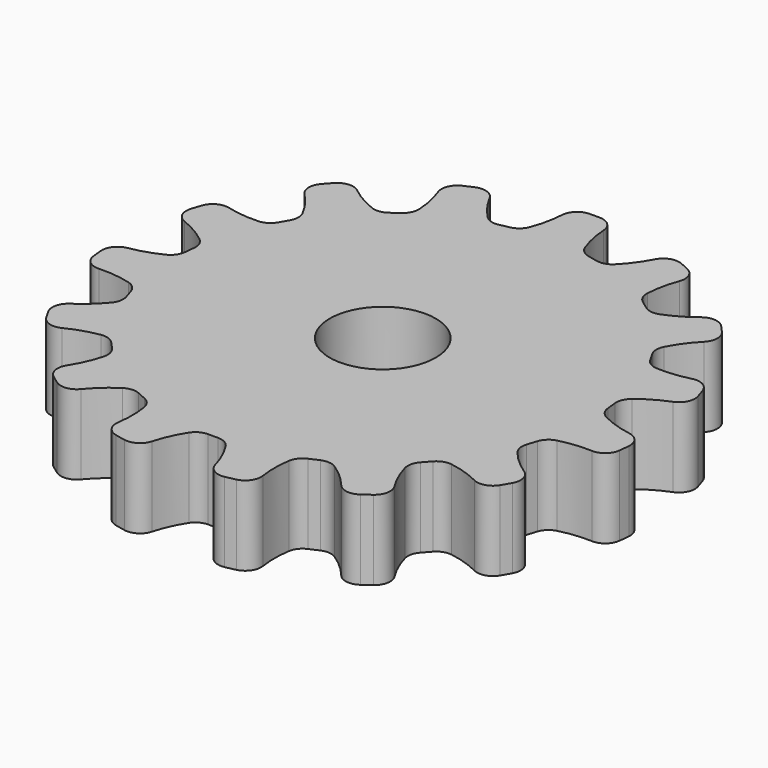
from build123d import *

# Parameters (mm, degrees)
F0_R            = 50
F1_DEPTH        = 15
F3_DEPTH        = 25
F3_COPIES_COUNT = 15
F4_R            = 3
F5_R            = 10
F6_DEPTH        = 25


# Not quite as in the source:
# - a pattern or mirror of a feature is missing from the dataset's text; its kind, count and spacing are read off the source's solid


with BuildPart() as f1:
    # F0 (on Top) → F1 (new body)
    with BuildSketch(Plane.XY):
        Circle(F0_R)
    extrude(amount=F1_DEPTH)

    # F2 (on face) → F3 (cut)
    with BuildSketch(Plane.XY.offset(15)):
        with BuildLine():
            ThreePointArc((-6.5, -49.5756996925), (0, -50), (6.5, -49.5756996925))
            ThreePointArc((6.5, -49.5756996925), (5.4393021929, -45.3055560091), (3.4705603608, -41.3706783092))
            ThreePointArc((3.4705603608, -41.3706783092), (2.3854522756, -40.3648562589), (0.9515703196, -40))
            Line((0.9515703196, -40), (-0.9515703196, -40))
            ThreePointArc((-0.9515703196, -40), (-2.3854522756, -40.3648562589), (-3.4705603608, -41.3706783092))
            ThreePointArc((-3.4705603608, -41.3706783092), (-5.4393021929, -45.3055560091), (-6.5, -49.5756996925))
        make_face()
    f3 = extrude(amount=-F3_DEPTH, mode=Mode.SUBTRACT)

    # F3_copies: F3 ×15 about axis
    f3_copies_axis = Axis((0, 0, 0), (0, 0, 1))
    for i in range(1, F3_COPIES_COUNT):
        add(f3.rotate(f3_copies_axis, i * 360 / F3_COPIES_COUNT), mode=Mode.SUBTRACT)

    # F4
    f4_edges = [f1.edges().sort_by_distance(p)[0] for p in [
        (14.226208, -47.933443, 7.5),
        (6.5, -49.5757, 7.5),
        (-6.5, -49.5757, 7.5),
        (-14.226208, -47.933443, 7.5),
        (-26.102299, -42.645867, 7.5),
        (-32.492576, -38.003059, 7.5),
        (-41.191274, -28.342177, 7.5),
        (-45.140682, -21.501601, 7.5),
        (-49.157903, -9.137866, 7.5),
        (-49.983554, -1.282321, 7.5),
        (-48.624684, 11.646464, 7.5),
        (-46.183815, 19.158685, 7.5),
        (-39.683815, 30.417015, 7.5),
        (-34.398476, 36.286979, 7.5),
        (-23.881255, 43.928188, 7.5),
        (-16.665327, 47.140926, 7.5),
        (-3.949408, 49.843778, 7.5),
        (3.949408, 49.843778, 7.5),
        (16.665327, 47.140926, 7.5),
        (23.881255, 43.928188, 7.5),
        (34.398476, 36.286979, 7.5),
        (39.683815, 30.417015, 7.5),
        (46.183815, 19.158685, 7.5),
        (48.624684, 11.646464, 7.5),
        (49.983554, -1.282321, 7.5),
        (49.157903, -9.137866, 7.5),
        (45.140682, -21.501601, 7.5),
        (41.191274, -28.342177, 7.5),
        (32.492576, -38.003059, 7.5),
        (26.102299, -42.645867, 7.5),
    ]]
    fillet(f4_edges, radius=F4_R)

    # F5 (on face) → F6 (cut)
    with BuildSketch(Plane.XY.offset(15)):
        Circle(F5_R)
    extrude(amount=-F6_DEPTH, mode=Mode.SUBTRACT)


solid = f1.part
